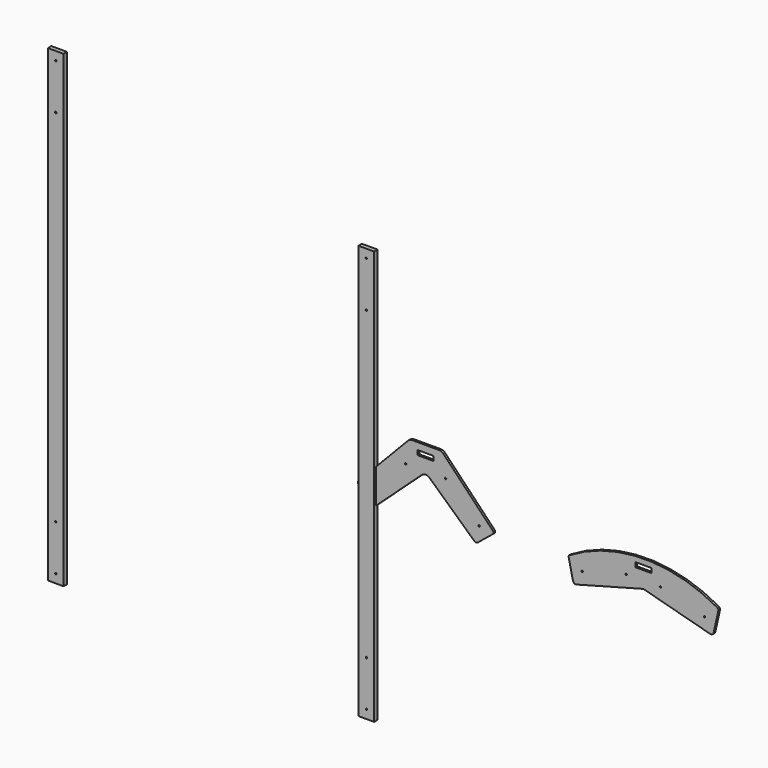
from build123d import *

# Parameters (mm, degrees)
F0_R     = 3.1877
F0_W     = 71.12
F0_H     = 20.32
F1_DEPTH = 9.525
F2_R     = 3.1877
F2_W     = 71.12
F2_H     = 20.32
F3_DEPTH = 9.525
F0_W_2   = 69.85
F0_H_2   = 2088.769
F4_DEPTH = 19.05
F0_H_3   = 1845.2592


# Not quite as in the source:
# - a length typed as a fraction of an inch, garbled in the dataset ("3 / 203.2 mm" for 3/8 in), is restored


with BuildPart() as f1:
    # F0 (on Front) → F1 (new body)
    with BuildSketch(Plane.XZ):
        with BuildLine():
            ThreePointArc((839.6723722923, 24.1515339259), (838.0317131921, 19.644837613), (838.1793448674, 14.8510626048))
            Line((838.1793448674, 14.8510626048), (857.2836977415, -70.2823224184))
            ThreePointArc((857.2836977415, -70.2823224184), (863.1011199006, -78.3674132665), (872.9625206832, -79.7687944446))
            Line((872.9625206832, -79.7687944446), (1167.3767125361, -0.8807494973))
            ThreePointArc((1167.3767125361, -0.8807494973), (1170.6637144089, -0.4480074912), (1173.9507162817, -0.8807494973))
            Line((1173.9507162817, -0.8807494973), (1468.3649081346, -79.7687944446))
            ThreePointArc((1468.3649081346, -79.7687944446), (1478.2263089171, -78.3674132665), (1484.0437310762, -70.2823224184))
            Line((1484.0437310762, -70.2823224184), (1504.5883732454, 21.2693225641))
            ThreePointArc((1504.5883732454, 21.2693225641), (1504.2165188216, 28.1501575378), (1500.3059571794, 33.8239281792))
            ThreePointArc((1500.3059571794, 33.8239281792), (1168.6711535979, 119.0091259816), (839.6723722923, 24.1515339259))
        make_face()
        with Locations((898.1589318866, -20.4254064456)):
            Circle(F0_R, mode=Mode.SUBTRACT)
        with Locations((1094.4350597885, 32.1666235192)):
            Circle(F0_R, mode=Mode.SUBTRACT)
        with Locations((1246.8923690293, 32.1666235192)):
            Circle(F0_R, mode=Mode.SUBTRACT)
        with Locations((1443.1684969312, -20.4254064456)):
            Circle(F0_R, mode=Mode.SUBTRACT)
        with Locations((1170.6637144089, 83.5188999772)):
            Rectangle(F0_W, F0_H, mode=Mode.SUBTRACT)
    extrude(amount=F1_DEPTH)


with BuildPart() as f3:
    # F2 (on Front) → F3 (new body)
    with BuildSketch(Plane.XZ):
        with BuildLine():
            ThreePointArc((-101.1592128677, 7.7226741622), (-100.7680553509, 0.798604341), (-96.7978449984, -4.8876226022))
            Line((-96.7978449984, -4.8876226022), (-32.5961750252, -57.3083489018))
            ThreePointArc((-32.5961750252, -57.3083489018), (-24.2017892971, -60.1658271529), (-15.9839681804, -56.8344145691))
            Line((-15.9839681804, -56.8344145691), (183.4770895885, 125.9379706671))
            ThreePointArc((183.4770895885, 125.9379706671), (200.6370808619, 132.6111263121), (217.7970721354, 125.9379706671))
            Line((217.7970721354, 125.9379706671), (417.2581299043, -56.8344145691))
            ThreePointArc((417.2581299043, -56.8344145691), (425.4759510209, -60.1658271529), (433.8703367491, -57.3083489018))
            Line((433.8703367491, -57.3083489018), (498.0720067222, -4.8876226022))
            ThreePointArc((498.0720067222, -4.8876226022), (502.0422170747, 0.798604341), (502.4333745915, 7.7226741622))
            Line((502.4333745915, 7.7226741622), (278.9733440379, 240.6731787355))
            ThreePointArc((278.9733440379, 240.6731787355), (270.6069010187, 246.4541627355), (260.6433282158, 248.4899333025))
            Line((260.6433282158, 248.4899333025), (200.6370808619, 248.4899333025))
            Line((200.6370808619, 248.4899333025), (140.6308335081, 248.4899333025))
            ThreePointArc((140.6308335081, 248.4899333025), (130.6672607051, 246.4541627355), (122.3008176859, 240.6731787355))
            Line((122.3008176859, 240.6731787355), (-101.1592128677, 7.7226741622))
        make_face()
        with Locations((-38.0776739779, 9.0481323209)):
            Circle(F2_R, mode=Mode.SUBTRACT)
        with Locations((111.7370808619, 146.3280625084)):
            Circle(F2_R, mode=Mode.SUBTRACT)
        with Locations((439.3518357017, 9.0481323209)):
            Circle(F2_R, mode=Mode.SUBTRACT)
        with Locations((289.5370808619, 146.3280625084)):
            Circle(F2_R, mode=Mode.SUBTRACT)
        with Locations((200.637060461, 207.5467059735)):
            Rectangle(F2_W, F2_H, mode=Mode.SUBTRACT)
    extrude(amount=F3_DEPTH)


with BuildPart() as f4:
    # F0 (on Front) → F4 (new body)
    with BuildSketch(Plane.XZ):
        with Locations((-1439.7445756912, 220.7827176781)):
            Rectangle(F0_W_2, F0_H_2)
        with Locations((-1439.7445756912, -785.5017823219)):
            Circle(F0_R, mode=Mode.SUBTRACT)
        with Locations((-1439.7445756912, -582.3017823219)):
            Circle(F0_R, mode=Mode.SUBTRACT)
        with Locations((-1439.7445756912, 1023.8672176781)):
            Circle(F0_R, mode=Mode.SUBTRACT)
        with Locations((-1439.7445756912, 1227.0672176781)):
            Circle(F0_R, mode=Mode.SUBTRACT)
    extrude(amount=F4_DEPTH)


with BuildPart() as f4b:
    # F0 (on Front) → F4, piece 2 (new body)
    with BuildSketch(Plane.XZ):
        with Locations((-56.0417547822, 17.06318371)):
            Rectangle(F0_W_2, F0_H_3)
        with Locations((-55.4067566991, -867.46641629)):
            Circle(F0_R, mode=Mode.SUBTRACT)
        with Locations((-55.4067566991, -664.26641629)):
            Circle(F0_R, mode=Mode.SUBTRACT)
        with Locations((-56.0417547822, 698.39278371)):
            Circle(F0_R, mode=Mode.SUBTRACT)
        with Locations((-56.0417547822, 901.59278371)):
            Circle(F0_R, mode=Mode.SUBTRACT)
    extrude(amount=F4_DEPTH)


solid = Compound([f1.part, f3.part, f4.part, f4b.part])
